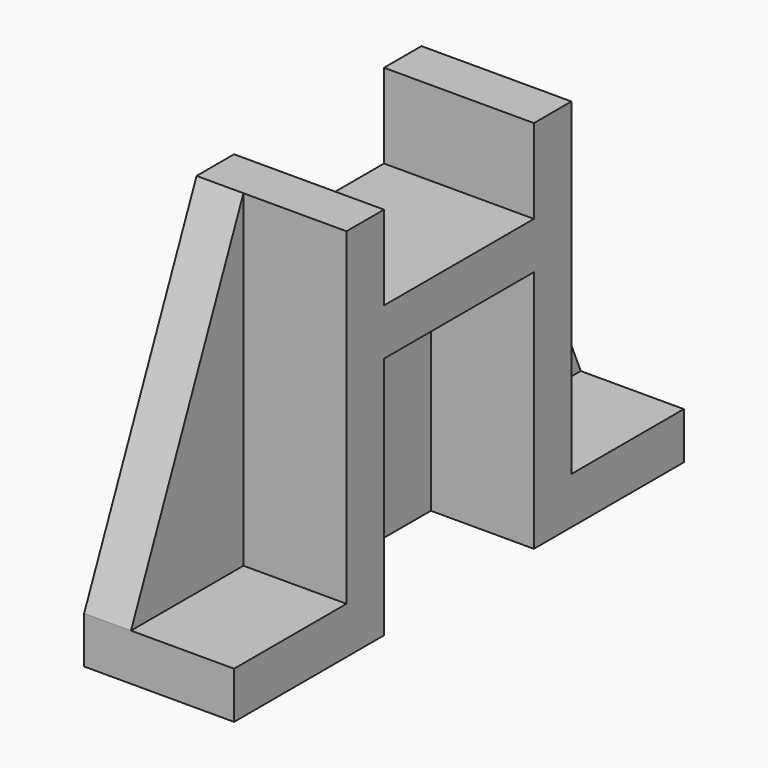
from build123d import *

# Parameters (mm, degrees)
F0_W     = 120
F0_H     = 80
F1_DEPTH = 32
F2_W     = 40
F2_H     = 52
F3_DEPTH = 22
F4_W     = 40
F4_H     = 18
F5_DEPTH = 32.001
F6_W     = 30
F6_H     = 70
F7_DEPTH = 32.001
F9_DEPTH = 10


# Not quite as in the source:
# - a pattern or mirror of a feature is missing from the dataset's text; its kind, count and spacing are read off the source's solid


with BuildPart() as f1:
    # F0 (on Right) → F1 (new body)
    with BuildSketch(Plane.YZ):
        Rectangle(F0_W, F0_H)
    extrude(amount=-F1_DEPTH)

    # F2 (on face) → F3 (cut)
    with BuildSketch(Plane.YZ):
        with Locations((0, -14)):
            Rectangle(F2_W, F2_H)
    extrude(amount=-F3_DEPTH, mode=Mode.SUBTRACT)

    # F4 (on face) → F5 (cut, through all)
    with BuildSketch(Plane.YZ):
        with Locations((0, 31)):
            Rectangle(F4_W, F4_H)
    extrude(amount=-F5_DEPTH, mode=Mode.SUBTRACT)

    # F6 (on face) → F7 (cut, through all)
    with BuildSketch(Plane.YZ):
        with Locations((-45, 5)):
            Rectangle(F6_W, F6_H)
    f7 = extrude(amount=-F7_DEPTH, mode=Mode.SUBTRACT)

    # F7_copies: F7 across plane
    add(f7.mirror(Plane.ZX), mode=Mode.SUBTRACT)

    # F8 (on face) → F9 (join)
    with BuildSketch(Plane(origin=(-32, 0, 0), x_dir=(0, -1, 0), z_dir=(-1, 0, 0))):
        Polygon((60, -30), (30, 40), (30, -30), align=None)
    f9 = extrude(amount=-F9_DEPTH)

    # F9_copies: F9 across plane
    add(f9.mirror(Plane.ZX))


solid = f1.part
